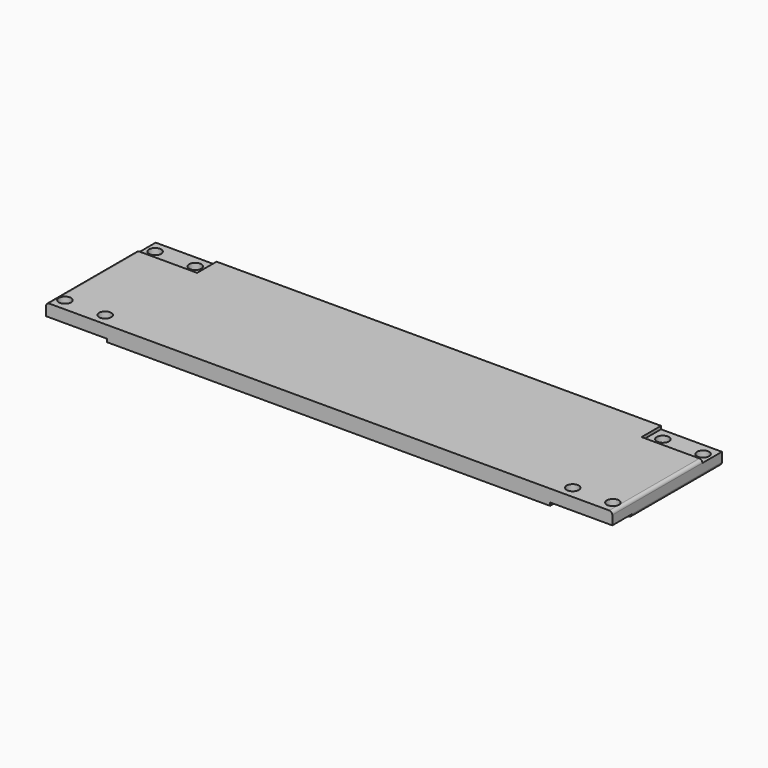
from build123d import *

# Parameters (mm, degrees)
F1_DEPTH  = 6.35
F2_W      = 25.4
F2_H      = 10.16
F3_DEPTH  = 1.27
F4_R      = 2.54
F5_DEPTH  = 25.4
F6_R      = 2.54
F7_DEPTH  = 25.4
F8_W      = 25.4
F8_H      = 10.16
F8_W_2    = 25.950329153
F9_DEPTH  = 1.27
F10_R     = 2.54
F11_DEPTH = 25.4
F12_R     = 2.54
F13_DEPTH = 25.4
F14_R     = 1.26999


# Not quite as in the source:
# - a fillet or chamfer is up to 0.001 mm smaller than in the source, because OpenCascade refuses the exact size


with BuildPart() as f1:
    # F0 (on Top) → F1 (new body)
    with BuildSketch(Plane.XY):
        Polygon((-53.3815915518, 5.5359576059), (-101.6415915518, 5.5359576059), (-101.6415915518, -51.6140423941), (-53.3815915518, -51.6140423941), (86.3184084482, -51.6140423941), (134.5784084482, -51.6140423941), (134.5784084482, 5.5359576059), (86.3184084482, 5.5359576059), align=None)
    extrude(amount=F1_DEPTH)

    # F2 (on face) → F3 (cut)
    with BuildSketch(Plane.XY.offset(6.35)):
        with Locations((-88.9415915518, 0.4559576059)):
            Rectangle(F2_W, F2_H)
        with Locations((121.8784084482, 0.4559576059)):
            Rectangle(F2_W, F2_H)
    extrude(amount=-F3_DEPTH, mode=Mode.SUBTRACT)

    # F4 (on face) → F5 (cut)
    with BuildSketch(Plane.XY.offset(5.08)):
        with Locations((-97.8315915518, 0.4559576059)):
            Circle(F4_R)
        with Locations((-81.0675915518, 0.4559576059)):
            Circle(F4_R)
    extrude(amount=-F5_DEPTH, mode=Mode.SUBTRACT)

    # F6 (on face) → F7 (cut)
    with BuildSketch(Plane.XY.offset(5.08)):
        with Locations((130.7684084482, 0.4559576059)):
            Circle(F6_R)
        with Locations((114.0044084482, 0.4559576059)):
            Circle(F6_R)
    extrude(amount=-F7_DEPTH, mode=Mode.SUBTRACT)

    # F8 (on face) → F9 (cut)
    with BuildSketch(Plane(origin=(0, 0, 0), x_dir=(1, 0, 0), z_dir=(0, 0, -1))):
        with Locations((-88.9415915518, 46.5340423941)):
            Rectangle(F8_W, F8_H)
        with Locations((121.6032438717, 46.5340423941)):
            Rectangle(F8_W_2, F8_H)
    extrude(amount=-F9_DEPTH, mode=Mode.SUBTRACT)

    # F10 (on face) → F11 (cut)
    with BuildSketch(Plane(origin=(0, 0, 1.27), x_dir=(1, 0, 0), z_dir=(0, 0, -1))):
        with Locations((-97.8315915518, 46.5340423941)):
            Circle(F10_R)
        with Locations((-81.0675915518, 46.5340423941)):
            Circle(F10_R)
    extrude(amount=-F11_DEPTH, mode=Mode.SUBTRACT)

    # F12 (on face) → F13 (cut)
    with BuildSketch(Plane(origin=(0, 0, 1.27), x_dir=(1, 0, 0), z_dir=(0, 0, -1))):
        with Locations((114.0044084482, 46.5340423941)):
            Circle(F12_R)
        with Locations((130.7684084482, 46.5340423941)):
            Circle(F12_R)
    extrude(amount=-F13_DEPTH, mode=Mode.SUBTRACT)

    # F14 (radius 1.27 in the source; OpenCascade refuses exactly that, so slightly less here)
    f14_edges = [f1.edges().sort_by_distance(p)[0] for p in [
        (134.578408, -28.119042, 6.35),
        (134.578408, -17.959042, 0),
        (-101.641592, -28.119042, 6.35),
        (-101.641592, -17.959042, 0),
    ]]
    fillet(f14_edges, radius=F14_R)


solid = f1.part
